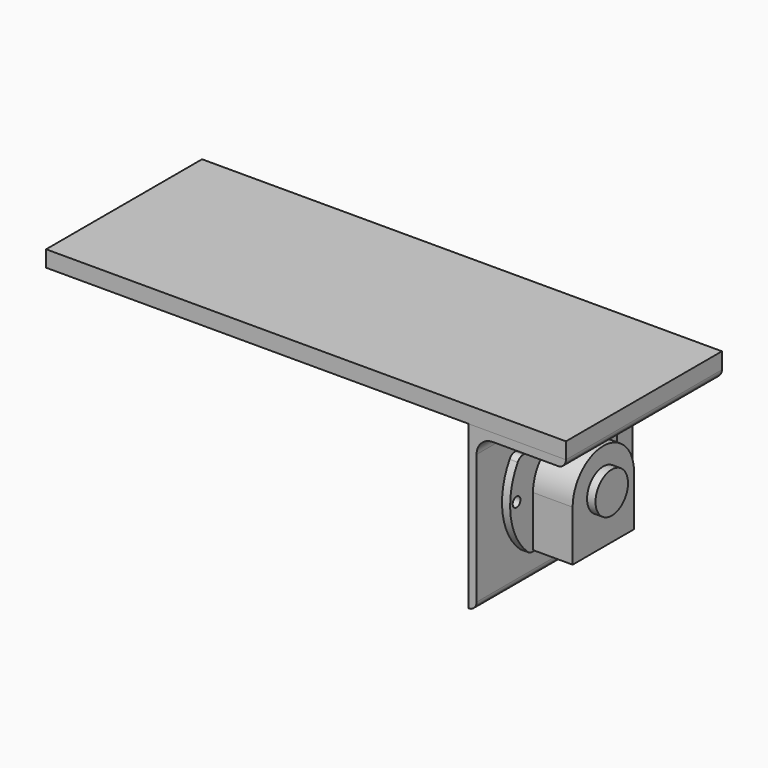
from build123d import *

# Parameters (mm, degrees)
F0_R            = 7.9375
F1_DEPTH        = 3.302
F2_DEPTH        = 15.494
F3_R            = 1.905
F3_R_2          = 3.175
F4_DEPTH        = 3.175
F5_R            = 3.175
F6_DEPTH        = 19.558
F5_R_2          = 6.35
F7_DEPTH        = 0.508
F8_R            = 3.175
F11_DEPTH       = 76.2
F12_R           = 3.17499
F13_R           = 6.35
F14_R           = 7.1628
F14_R_2         = 1.016
F15_DEPTH       = 25.4
F17_W           = 203.2
F17_H           = 76.2
F18_DEPTH       = 6.35
F20_D           = 4.2926
F20_DEPTH       = 19.05
F20_CSINK_D     = 9.525
F20_CSINK_ANGLE = 82
F20_TIP         = 1.2896271466


# Not quite as in the source:
# - a fillet or chamfer is up to 0.001 mm smaller than in the source, because OpenCascade refuses the exact size


with BuildPart() as f1:
    # F0 (on Right) → F1 (new body)
    with BuildSketch(Plane.YZ):
        Circle(F0_R)
    extrude(amount=F1_DEPTH)

    # F0 (on Right) → F2 (join)
    with BuildSketch(Plane.YZ):
        with BuildLine():
            ThreePointArc((-14.986, 0), (0, -14.986), (14.986, 0))
            ThreePointArc((14.986, 0), (0, 14.986), (-14.986, 0))
        make_face()
        Circle(F0_R, mode=Mode.SUBTRACT)
        with BuildLine():
            Line((14.986, -19.812), (14.986, 0))
            ThreePointArc((14.986, 0), (0, -14.986), (-14.986, 0))
            Line((-14.986, 0), (-14.986, -19.812))
            Line((-14.986, -19.812), (14.986, -19.812))
        make_face()
        Circle(F0_R)
    extrude(amount=-F2_DEPTH)

    # F3 (on face) → F4 (join)
    with BuildSketch(Plane(origin=(-15.494, 0, 0), x_dir=(0, -1, 0), z_dir=(-1, 0, 0))):
        with BuildLine():
            Line((-2.18e-08, 14.986), (-21.4445808539, 14.986))
            ThreePointArc((-21.4445808539, 14.986), (-25.9069948799, -3.6438798406), (-16.4787088086, -20.32))
            Line((-16.4787088086, -20.32), (16.4787088086, -20.32))
            ThreePointArc((16.4787088086, -20.32), (25.9069948799, -3.6438798406), (21.4445808539, 14.986))
            Line((21.4445808539, 14.986), (-2.18e-08, 14.986))
        make_face()
        with Locations((-23.0124, 0)):
            Circle(F3_R, mode=Mode.SUBTRACT)
        with BuildLine():
            ThreePointArc((-14.986, 0), (-10.5967022306, 10.5967022152), (-2.18e-08, 14.986))
            ThreePointArc((-2.18e-08, 14.986), (10.5967022152, 10.5967022306), (14.986, 0))
            Line((14.986, 0), (14.986, -19.812))
            Line((14.986, -19.812), (-14.986, -19.812))
            Line((-14.986, -19.812), (-14.986, 0))
        make_face(mode=Mode.SUBTRACT)
        with Locations((23.0124, 0)):
            Circle(F3_R, mode=Mode.SUBTRACT)
        with BuildLine():
            ThreePointArc((14.986, 0), (10.5967022152, 10.5967022306), (-2.18e-08, 14.986))
            ThreePointArc((-2.18e-08, 14.986), (-10.5967022306, 10.5967022152), (-14.986, 0))
            Line((-14.986, 0), (-14.986, -19.812))
            Line((-14.986, -19.812), (14.986, -19.812))
            Line((14.986, -19.812), (14.986, 0))
        make_face()
        Circle(F3_R_2, mode=Mode.SUBTRACT)
        Circle(F3_R_2)
    extrude(amount=F4_DEPTH)

    # F5 (on face) → F6 (join)
    with BuildSketch(Plane(origin=(-18.669, 0, 0), x_dir=(0, -1, 0), z_dir=(-1, 0, 0))):
        Circle(F5_R)
    extrude(amount=F6_DEPTH)

    # F5 (on face) → F7 (join)
    with BuildSketch(Plane(origin=(-18.669, 0, 0), x_dir=(0, -1, 0), z_dir=(-1, 0, 0))):
        Circle(F5_R_2)
        Circle(F5_R, mode=Mode.SUBTRACT)
    extrude(amount=F7_DEPTH)

    # F8
    f8_edges = [f1.edges().sort_by_distance(p)[0] for p in [
        (-17.0815, -21.444581, 14.986),
        (-17.0815, 21.444581, 14.986),
        (-17.0815, 16.478709, -20.32),
        (-17.0815, -16.478709, -20.32),
    ]]
    fillet(f8_edges, radius=F8_R)


with BuildPart() as f11:
    # F10 (on offset) → F11 (new body)
    with BuildSketch(Plane.XZ.offset(38.1)):
        Polygon((-22.225, 30.861), (-22.225, -32.639), (-19.05, -32.639), (-19.05, 27.686), (15.875, 27.686), (15.875, 30.861), align=None)
    extrude(amount=-F11_DEPTH)

    # F12 (radius 3.175 in the source; OpenCascade refuses exactly that, so slightly less here)
    f12_edges = [f11.edges().sort_by_distance(p)[0] for p in [
        (15.875, 0, 27.686),
        (-19.05, 0, -32.639),
    ]]
    fillet(f12_edges, radius=F12_R)

    # F13
    f13_edges = [f11.edges().sort_by_distance(p)[0] for p in [
        (-19.05, 0, 27.686),
    ]]
    fillet(f13_edges, radius=F13_R)

    # F14 (on face) → F15 (cut)
    with BuildSketch(Plane(origin=(-22.225, 0, 0), x_dir=(0, -1, 0), z_dir=(-1, 0, 0))):
        Circle(F14_R)
        with Locations((23.0124, 0)):
            Circle(F14_R_2)
        with Locations((-23.0124, 0)):
            Circle(F14_R_2)
    extrude(amount=-F15_DEPTH, mode=Mode.SUBTRACT)

    # F20
    with Locations(Plane(origin=(0, 0, 27.686), x_dir=(1, 0, 0), z_dir=(0, 0, -1))):
        with Locations((0, -25.4), (0, 25.4)):
            CounterSinkHole(F20_D / 2, F20_CSINK_D / 2, depth=F20_DEPTH, counter_sink_angle=F20_CSINK_ANGLE)
            with Locations((0, 0, -(F20_DEPTH + F20_TIP / 2))):  # 118° drill point
                Cone(0, F20_D / 2, F20_TIP, mode=Mode.SUBTRACT)


with BuildPart() as f18:
    # F17 (on face) → F18 (new body)
    with BuildSketch(Plane.XY.offset(30.861)):
        with Locations((-85.725, 0)):
            Rectangle(F17_W, F17_H)
    extrude(amount=F18_DEPTH)


solid = Compound([f1.part, f11.part, f18.part])
